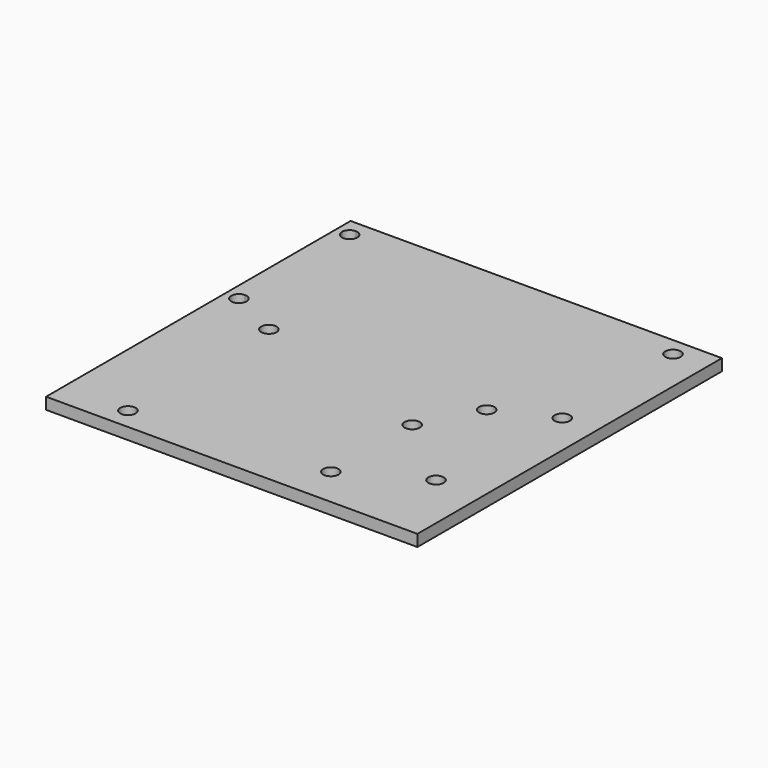
from build123d import *

# Parameters (mm, degrees)
F0_R     = 2.0955
F1_DEPTH = 3.175


with BuildPart() as f1:
    # F0 (on Top) → F1 (new body)
    with BuildSketch(Plane.XY):
        with BuildLine():
            Line((3.81, 0), (0, 0))
            Line((0, 0), (0, -5.08))
            Line((0, -5.08), (1.7145, -5.08))
            ThreePointArc((1.7145, -5.08), (2.32825774, -3.59825774), (3.81, -2.9845))
            Line((3.81, -2.9845), (3.81, 0))
        make_face()
        with BuildLine():
            Line((101.6, 0), (3.81, 0))
            Line((3.81, 0), (3.81, -2.9845))
            ThreePointArc((3.81, -2.9845), (5.29174226, -3.59825774), (5.9055, -5.08))
            Line((5.9055, -5.08), (90.1827, -5.08))
            ThreePointArc((90.1827, -5.08), (92.2782, -2.9845), (94.3737, -5.08))
            Line((94.3737, -5.08), (101.6, -5.08))
            Line((101.6, -5.08), (101.6, 0))
        make_face()
        with BuildLine():
            Line((1.7145, -5.08), (0, -5.08))
            Line((0, -5.08), (0, -104.14))
            Line((0, -104.14), (3.81, -104.14))
            Line((3.81, -104.14), (3.81, -50.0634))
            Line((3.81, -50.0634), (3.81, -45.0469))
            ThreePointArc((3.81, -45.0469), (1.7145, -42.9514), (3.81, -40.8559))
            Line((3.81, -40.8559), (3.81, -7.1755))
            ThreePointArc((3.81, -7.1755), (2.32825774, -6.56174226), (1.7145, -5.08))
        make_face()
        with BuildLine():
            Line((101.6, -104.14), (101.6, -5.08))
            Line((101.6, -5.08), (94.3737, -5.08))
            ThreePointArc((94.3737, -5.08), (92.2782, -7.1755), (90.1827, -5.08))
            Line((90.1827, -5.08), (5.9055, -5.08))
            ThreePointArc((5.9055, -5.08), (5.29174226, -6.56174226), (3.81, -7.1755))
            Line((3.81, -7.1755), (3.81, -40.8559))
            ThreePointArc((3.81, -40.8559), (5.29174226, -41.46965774), (5.9055, -42.9514))
            ThreePointArc((5.9055, -42.9514), (5.29174226, -44.43314226), (3.81, -45.0469))
            Line((3.81, -45.0469), (3.81, -50.0634))
            Line((3.81, -50.0634), (3.81, -104.14))
            Line((3.81, -104.14), (101.6, -104.14))
        make_face()
        with Locations((17.7038, -98.2599)):
            Circle(F0_R, mode=Mode.SUBTRACT)
        with Locations((69.215, -93.2561)):
            Circle(F0_R, mode=Mode.SUBTRACT)
        with Locations((89.154, -82.2198)):
            Circle(F0_R, mode=Mode.SUBTRACT)
        with Locations((69.215, -65.4431)):
            Circle(F0_R, mode=Mode.SUBTRACT)
        with BuildLine():
            ThreePointArc((19.7993, -50.0634), (17.7038, -52.1589), (15.6083, -50.0634))
            ThreePointArc((15.6083, -50.0634), (17.7038, -47.9679), (19.7993, -50.0634))
        make_face(mode=Mode.SUBTRACT)
        with BuildLine():
            ThreePointArc((79.3877, -50.0634), (77.2922, -52.1589), (75.1967, -50.0634))
            ThreePointArc((75.1967, -50.0634), (77.2922, -47.9679), (79.3877, -50.0634))
        make_face(mode=Mode.SUBTRACT)
        with BuildLine():
            ThreePointArc((94.3737, -42.9514), (92.2782, -45.0469), (90.1827, -42.9514))
            ThreePointArc((90.1827, -42.9514), (92.2782, -40.8559), (94.3737, -42.9514))
        make_face(mode=Mode.SUBTRACT)
    extrude(amount=-F1_DEPTH)


solid = f1.part
